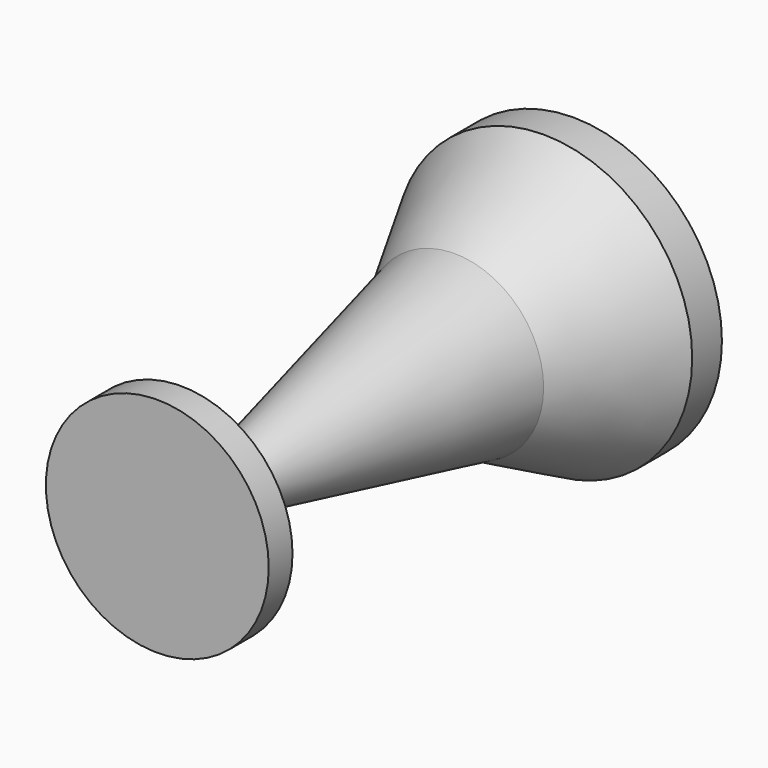
from build123d import *

# Parameters (mm, degrees)
F0_W      = 25.4
F0_H      = 25.4
F2_SIZE2  = 19.05
F2_SIZE   = 10.16
F3_W      = 7.62
F3_H      = 6.35
F3_W_2    = 6.35
F3_H_2    = 7.62
F4_DEPTH  = 12.7
F5_SIZE2  = 12.69999
F5_SIZE   = 7.61999
F6_R      = 2.54
F7_R      = 15.24
F8_DEPTH  = 63.5
F9_SIZE2  = 63.49999
F9_SIZE   = 13.96999
F10_R     = 19.05
F10_R_2   = 1.27001
F11_DEPTH = 5.08


# Not quite as in the source:
# - a fillet or chamfer is up to 0.001 mm smaller than in the source, because OpenCascade refuses the exact size


with BuildPart() as f1:
    # F0 (on Top) → F1 (revolve)
    with BuildSketch(Plane.XY):
        Rectangle(F0_W, F0_H)
    revolve(axis=Axis((-12.7, 0, 0), (0, 1, 0)))

    # F2
    f2_edges = [f1.edges().sort_by_distance(p)[0] for p in [
        (-38.1, -12.7, 0),
    ]]
    chamfer(f2_edges, length=F2_SIZE, length2=F2_SIZE2)

    # F3 (on face) → F4 (cut, symmetric)
    with BuildSketch(Plane(origin=(0, 12.7, 0), x_dir=(-1, 0, 0), z_dir=(0, 1, 0))):
        with Locations((12.7, 6.985)):
            Rectangle(F3_W, F3_H)
        with Locations((5.715, 0)):
            Rectangle(F3_W_2, F3_H_2)
        with Locations((12.7, 0)):
            Rectangle(F3_W, F3_H_2)
        with Locations((19.685, 0)):
            Rectangle(F3_W_2, F3_H_2)
        with Locations((12.7, -6.985)):
            Rectangle(F3_W, F3_H)
    extrude(amount=F4_DEPTH, both=True, mode=Mode.SUBTRACT)

    # F5 (size 7.62 and 12.7 in the source; OpenCascade refuses exactly that, so slightly less here)
    f5_edges = [f1.edges().sort_by_distance(p)[0] for p in [
        (-12.7, 12.7, 10.16),
        (-2.54, 12.7, 0),
        (-22.86, 12.7, 0),
        (-12.7, 12.7, -10.16),
    ]]
    chamfer(f5_edges, length=F5_SIZE, length2=F5_SIZE2)

    # F6
    f6_edges = [f1.edges().sort_by_distance(p)[0] for p in [
        (-8.89, 6.35, -3.81),
        (-16.51, 6.35, -3.81),
        (-8.89, 6.35, 3.81),
        (-16.51, 6.35, 3.81),
    ]]
    fillet(f6_edges, radius=F6_R)

    # F7 (on face) → F8 (join)
    with BuildSketch(Plane.XZ.offset(12.7)):
        with Locations((-12.7, 0)):
            Circle(F7_R)
    extrude(amount=F8_DEPTH)

    # F9 (size 13.97 and 63.5 in the source; OpenCascade refuses exactly that, so slightly less here)
    f9_edges = [f1.edges().sort_by_distance(p)[0] for p in [
        (-27.94, -76.2, 0),
    ]]
    f9_side = f1.faces().sort_by_distance((-12.7, -76.2, 0))[0]
    chamfer(f9_edges, length=F9_SIZE, length2=F9_SIZE2, reference=f9_side)

    # F10 (on face) → F11 (join)
    with BuildSketch(Plane.XZ.offset(76.2)):
        with Locations((-12.7, 0)):
            Circle(F10_R)
        with Locations((-12.7, 0)):
            Circle(F10_R_2, mode=Mode.SUBTRACT)
    extrude(amount=-F11_DEPTH)


solid = f1.part
